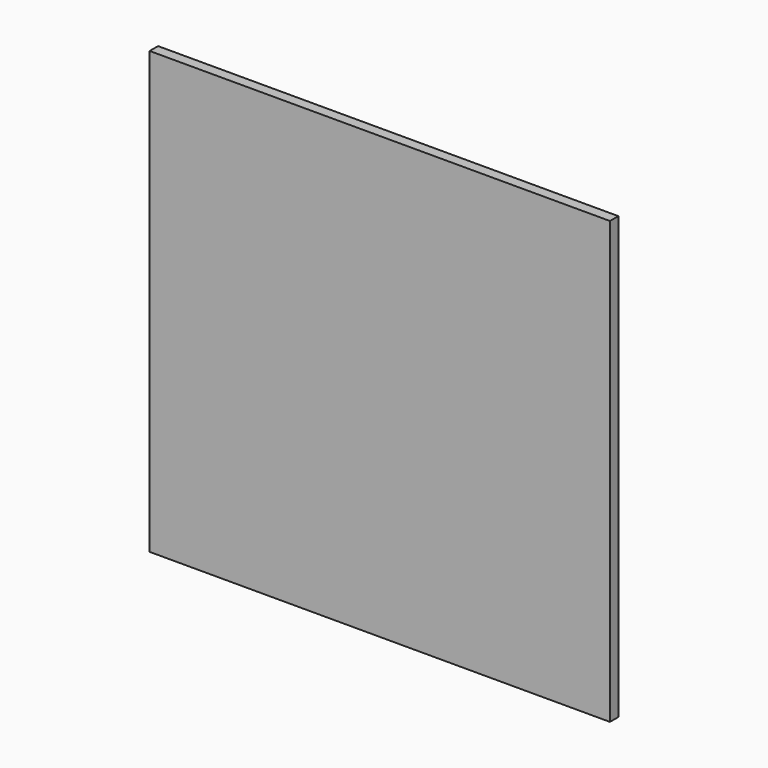
from build123d import *

# Parameters (mm, degrees)
F0_W      = 500
F0_H      = 500
F1_DEPTH  = 12
F2_W      = 500
F2_H      = 50
F3_DEPTH  = 6
F6_DEPTH  = 6
F14_DEPTH = 6
F15_R     = 19.99999
F19_DEPTH = 6
F22_DEPTH = 12
F25_DEPTH = 6
F27_W     = 12
F27_H     = 320
F28_DEPTH = 44
F31_W     = 196
F31_H     = 12
F32_DEPTH = 44
F37_DEPTH = 3
F43_DEPTH = 12


# Not quite as in the source:
# - a fillet or chamfer is up to 0.001 mm smaller than in the source, because OpenCascade refuses the exact size


with BuildPart() as f1:
    # F0 (on Top) → F1 (new body)
    with BuildSketch(Plane.XY):
        Rectangle(F0_W, F0_H)
    extrude(amount=F1_DEPTH)


with BuildPart() as f3:
    # F2 (on Right) → F3 (new body, symmetric)
    with BuildSketch(Plane.YZ):
        Rectangle(F2_W, F2_H)
    extrude(amount=F3_DEPTH, both=True)


with BuildPart() as f3_1:
    # F4: moved
    add(f3.part.moved(Location((0, 0, -25))))


with BuildPart() as f6:
    # F5 (on Front) → F6 (new body, symmetric)
    with BuildSketch(Plane.XZ):
        Polygon((-250, -25), (250, -25), (250, 25), (6, 25), (6, 0), (-6, 0), (-6, 25), (-250, 25), align=None)
    extrude(amount=F6_DEPTH, both=True)


with BuildPart() as f6_1:
    # F7: moved
    add(f6.part.moved(Location((0, 80, -25))))


with BuildPart() as f8_1:
    # F8: copy of F6
    add(f6_1.part)


with BuildPart() as f3_2:
    add(f3_1.part)

    # F10: cut F6
    add(f6_1.part, mode=Mode.SUBTRACT)


with BuildPart() as f11_1:
    # F11: copy of F6
    add(f6_1.part.moved(Location((0, 164, 0))))


with BuildPart() as f3_3:
    add(f3_2.part)

    # F12: cut F11_1
    add(f11_1.part, mode=Mode.SUBTRACT)


with BuildPart() as f14:
    # F13 (on Right) → F14 (new body, symmetric)
    with BuildSketch(Plane.YZ):
        Polygon((250, -50), (250, 0), (250, 452), (70, 452), (-110, 452), (-250, 100), (-250, -50), align=None)
        Polygon((0, 412), (70, 412), (140, 412), (140, 372), (0, 372), align=None, mode=Mode.SUBTRACT)
    extrude(amount=F14_DEPTH, both=True)

    # F15 (radius 20 in the source; OpenCascade refuses exactly that, so slightly less here)
    f15_edges = [f14.edges().sort_by_distance(p)[0] for p in [
        (0, 140, 372),
        (0, 140, 412),
        (0, 0, 412),
        (0, 0, 372),
    ]]
    fillet(f15_edges, radius=F15_R)


with BuildPart() as f14_1:
    # F16: moved
    add(f14.part.moved(Location((-256, 0, 0))))


with BuildPart() as f17_1:
    # F17: copy of F14
    add(f14_1.part.moved(Location((512, 0, 0))))


with BuildPart() as f19:
    # F18 (on Front) → F19 (new body, symmetric)
    with BuildSketch(Plane.XZ):
        Polygon((-262, 452), (-262, 0), (-262, -50), (262, -50), (262, 452), align=None)
    extrude(amount=F19_DEPTH, both=True)


with BuildPart() as f19_1:
    # F20: moved
    add(f19.part.moved(Location((0, 256, 0))))


with BuildPart() as f22:
    # F21 (on face) → F22 (new body)
    with BuildSketch(Plane.XY.offset(12)):
        Polygon((262, 262), (0, 262), (-262, 262), (-262, -110), (262, -110), align=None)
    extrude(amount=F22_DEPTH)


with BuildPart() as f22_1:
    # F23: moved
    add(f22.part.moved(Location((0, 0, 440))))


with BuildPart() as f25:
    # F24 (on Front) → F25 (new body, symmetric)
    with BuildSketch(Plane.XZ):
        Polygon((-250, 12), (0, 12), (250, 12), (250, 100), (-250, 100), align=None)
    extrude(amount=F25_DEPTH, both=True)


with BuildPart() as f25_1:
    # F26: moved
    add(f25.part.moved(Location((0, -244, 0))))


with BuildPart() as f28:
    # F27 (on Top) → F28 (new body)
    with BuildSketch(Plane.XY):
        with Locations((-24, -90)):
            Rectangle(F27_W, F27_H)
    extrude(amount=F28_DEPTH)


with BuildPart() as f28_1:
    # F29: moved
    add(f28.part.moved(Location((0, 0, -48))))


with BuildPart() as f30_1:
    # F30: copy of F28
    add(f28_1.part.moved(Location((-208, 0, 0))))


with BuildPart() as f32:
    # F31 (on Top) → F32 (new body)
    with BuildSketch(Plane.XY):
        with Locations((-128, -244)):
            Rectangle(F31_W, F31_H)
    extrude(amount=-F32_DEPTH)


with BuildPart() as f32_1:
    # F33: moved
    add(f32.part.moved(Location((0, 0, -4))))


with BuildPart() as f34_1:
    # F34: copy of F32
    add(f32_1.part.moved(Location((0, 308, 0))))


with BuildPart() as f35_1:
    # F35: copy of F32
    add(f32_1.part.moved(Location((256, 0, 0))))


with BuildPart() as f35_2:
    # F35: copy of F30_1
    add(f30_1.part.moved(Location((256, 0, 0))))


with BuildPart() as f35_3:
    # F35: copy of F28
    add(f28_1.part.moved(Location((256, 0, 0))))


with BuildPart() as f35_4:
    # F35: copy of F34_1
    add(f34_1.part.moved(Location((256, 0, 0))))


with BuildPart() as f37:
    # F36 (on Top) → F37 (new body)
    with BuildSketch(Plane.XY):
        Polygon((-24, -244), (-24, 0), (-24, 64), (-232, 64), (-232, -244), align=None)
    extrude(amount=F37_DEPTH)


with BuildPart() as f37_1:
    # F38: moved
    add(f37.part.moved(Location((0, 0, -44))))


with BuildPart() as f39_1:
    # F39: copy of F37
    add(f37_1.part.moved(Location((256, 0, 0))))


with BuildPart() as f30_1_1:
    add(f30_1.part)

    # F40: cut F37
    add(f37_1.part, mode=Mode.SUBTRACT)


with BuildPart() as f32_2:
    add(f32_1.part)

    # F40: cut F37
    add(f37_1.part, mode=Mode.SUBTRACT)


with BuildPart() as f28_2:
    add(f28_1.part)

    # F40: cut F37
    add(f37_1.part, mode=Mode.SUBTRACT)


with BuildPart() as f34_1_1:
    add(f34_1.part)

    # F40: cut F37
    add(f37_1.part, mode=Mode.SUBTRACT)


with BuildPart() as f35_1_1:
    add(f35_1.part)

    # F41: cut F39_1
    add(f39_1.part, mode=Mode.SUBTRACT)


with BuildPart() as f35_3_1:
    add(f35_3.part)

    # F41: cut F39_1
    add(f39_1.part, mode=Mode.SUBTRACT)


with BuildPart() as f35_4_1:
    add(f35_4.part)

    # F41: cut F39_1
    add(f39_1.part, mode=Mode.SUBTRACT)


with BuildPart() as f35_2_1:
    add(f35_2.part)

    # F41: cut F39_1
    add(f39_1.part, mode=Mode.SUBTRACT)


with BuildPart() as f43:
    # F42 (on Front) → F43 (new body)
    with BuildSketch(Plane.XZ):
        Polygon((0, 12), (0, 0), (0, -50), (262, -50), (262, 12), align=None)
    extrude(amount=F43_DEPTH)


with BuildPart() as f43_1:
    # F44: moved
    add(f43.part.moved(Location((0, -250, 0))))


with BuildPart() as f45_1:
    # F45: copy of F43
    add(f43_1.part.moved(Location((-262, 0, 0))))


solid = f19_1.part
